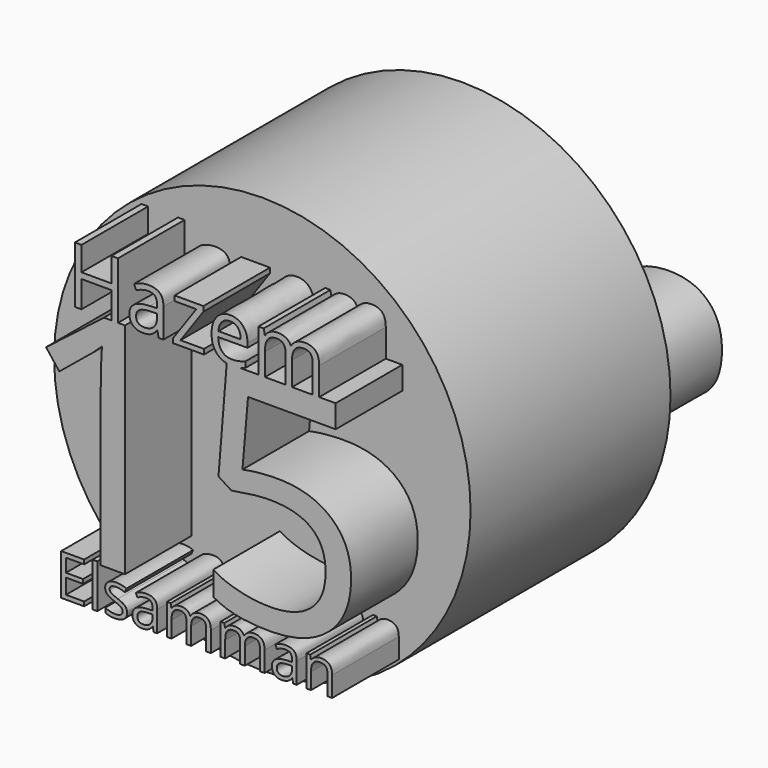
from build123d import *

# Parameters (mm, degrees)
F0_R         = 63.5
F1_DEPTH     = 76.2
F2_TEXT_SIZE = 93.5510697726
F3_DEPTH     = 25.4
F4_TEXT_SIZE = 24.2313608121
F5_DEPTH     = 25.4
F6_TEXT_SIZE = 17.601021579
F7_DEPTH     = 25.4
F8_TEXT_SIZE = 43.4321208416
F9_DEPTH     = 25.4


# Not quite as in the source:
# - Text() gives the source's letters only with a copy of the font that has no kerning and outlines rounded to 1/6400 em; it was checked with that copy


with BuildPart() as f1:
    # F0 (on Front) → F1 (new body)
    with BuildSketch(Plane.XZ):
        Circle(F0_R)
    extrude(amount=F1_DEPTH)

    # F2 (on face) → F3 (join)
    with BuildSketch(Plane.XZ.offset(76.2)):
        with Locations((-54.2104505281, -34.2890056679)):
            Text('15', F2_TEXT_SIZE, font='Open Sans', text_align=(TextAlign.LEFT, TextAlign.BOTTOM))
    extrude(amount=F3_DEPTH)

    # F4 (on face) → F5 (join)
    with BuildSketch(Plane.XZ.offset(76.2)):
        with Locations((-39.2150499392, 32.4976877369)):
            Text('Hazem', F4_TEXT_SIZE, font='Open Sans', text_align=(TextAlign.LEFT, TextAlign.BOTTOM))
    extrude(amount=F5_DEPTH)

    # F6 (on face) → F7 (join)
    with BuildSketch(Plane.XZ.offset(76.2)):
        with Locations((-42.7416057608, -46.9617412048)):
            Text('Elsamman', F6_TEXT_SIZE, font='Open Sans', text_align=(TextAlign.LEFT, TextAlign.BOTTOM))
    extrude(amount=F7_DEPTH)

    # F8 (on face) → F9 (join)
    with BuildSketch(Plane(origin=(0, 0, 0), x_dir=(-1, 0, 0), z_dir=(0, 1, 0))):
        with Locations((-61.3760780078, -14.9853341675)):
            Text('GOAT', F8_TEXT_SIZE, font='Open Sans', font_style=FontStyle.BOLD, text_align=(TextAlign.LEFT, TextAlign.BOTTOM))
    extrude(amount=F9_DEPTH)


solid = f1.part
